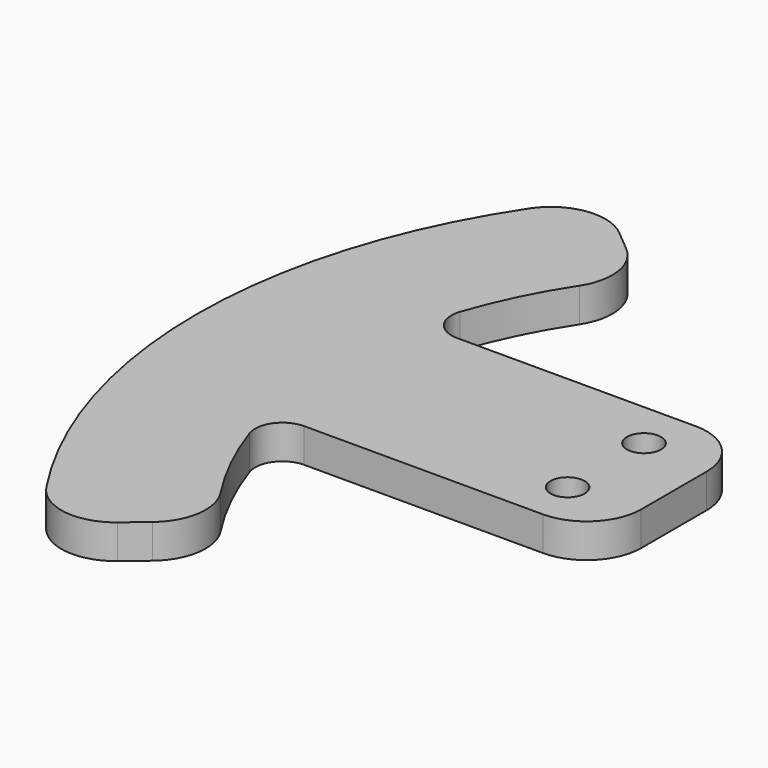
from build123d import *

# Parameters (mm, degrees)
F0_R     = 1.5875
F1_DEPTH = 3.175
F2_R     = 5.08
F3_R     = 5.08
F4_R     = 2.54
F5_R     = 5.08


with BuildPart() as f1:
    # F0 (on Top) → F1 (new body)
    with BuildSketch(Plane.XY):
        with BuildLine():
            ThreePointArc((-50.8, 0), (-47.7363851359, -17.3746232809), (-38.9150577104, -32.6536105721))
            Line((-38.9150577104, -32.6536105721), (-29.1862932828, -24.4902079291))
            ThreePointArc((-29.1862932828, -24.4902079291), (-34.023485561, -17.14679067), (-37.0483184504, -8.89))
            Line((-37.0483184504, -8.89), (-6.35, -8.89))
            Line((-6.35, -8.89), (-6.35, 0))
            Line((-6.35, 0), (-6.35, 8.89))
            Line((-6.35, 8.89), (-37.0483184504, 8.89))
            ThreePointArc((-37.0483184504, 8.89), (-34.023485561, 17.14679067), (-29.1862932828, 24.4902079291))
            Line((-29.1862932828, 24.4902079291), (-38.9150577104, 32.6536105721))
            ThreePointArc((-38.9150577104, 32.6536105721), (-47.7363851359, 17.3746232809), (-50.8, 0))
        make_face()
        with Locations((-12.7, -4.445)):
            Circle(F0_R, mode=Mode.SUBTRACT)
        with Locations((-12.7, 4.445)):
            Circle(F0_R, mode=Mode.SUBTRACT)
    extrude(amount=F1_DEPTH)

    # F2
    f2_edges = [f1.edges().sort_by_distance(p)[0] for p in [
        (-38.915058, 32.653611, 1.5875),
        (-38.915058, -32.653611, 1.5875),
    ]]
    fillet(f2_edges, radius=F2_R)

    # F3
    f3_edges = [f1.edges().sort_by_distance(p)[0] for p in [
        (-29.186293, 24.490208, 1.5875),
        (-29.186293, -24.490208, 1.5875),
    ]]
    fillet(f3_edges, radius=F3_R)

    # F4
    f4_edges = [f1.edges().sort_by_distance(p)[0] for p in [
        (-37.048318, -8.89, 1.5875),
        (-37.048318, 8.89, 1.5875),
    ]]
    fillet(f4_edges, radius=F4_R)

    # F5
    f5_edges = [f1.edges().sort_by_distance(p)[0] for p in [
        (-6.35, 8.89, 1.5875),
        (-6.35, -8.89, 1.5875),
    ]]
    fillet(f5_edges, radius=F5_R)


solid = f1.part
